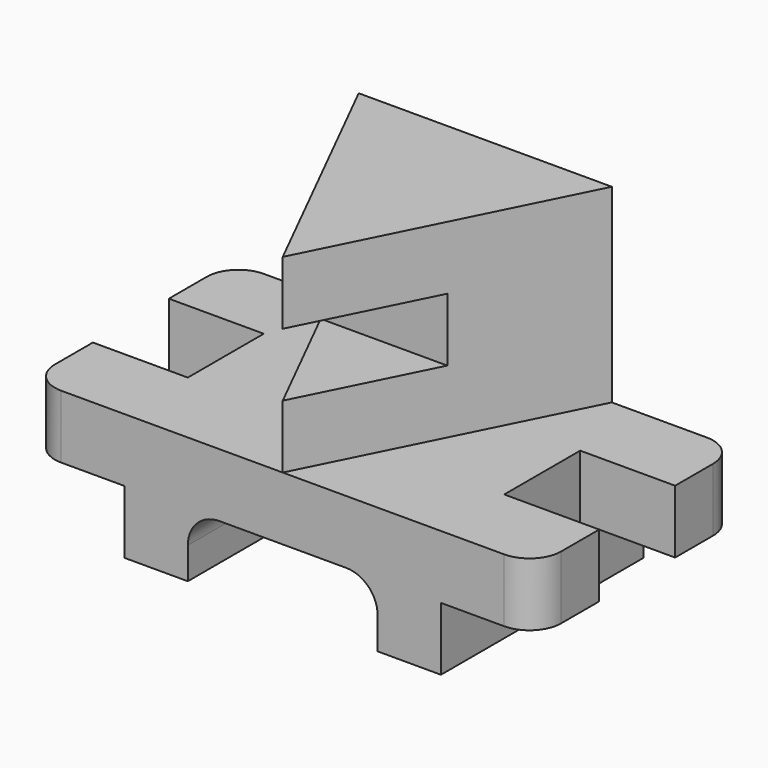
from build123d import *

# Parameters (mm, degrees)
F1_DEPTH       = 50.8
F2_W           = 76.2
F2_H           = 25.4
F3_DEPTH       = 101.601
F4_R           = 12.7
F5_R           = 12.7
F6_W           = 38.1
F6_H           = 25.4
F7_DEPTH       = 38.1
F8_W           = 38.1
F8_H           = 25.4
F9_DEPTH       = 38.1
F10_R          = 12.7
F11_W          = 101.6
F11_H          = 76.2
F12_DEPTH      = 50.8
F12_DEPTH_BACK = 50.8
F14_DEPTH      = 76.2
F15_W          = 50.8
F15_H          = 25.4
F16_DEPTH      = 101.601
F16_DEPTH_BACK = 356
F17_DEPTH      = 50.8


# Not quite as in the source:
# - an extrude ends at something that could not be found from the text; its depth is read off the source's solid


with BuildPart() as f1:
    # F0 (on Front) → F1 (new body, symmetric)
    with BuildSketch(Plane.XZ):
        Polygon((0, 25.4), (0, 0), (127, 0), (127, 25.4), (165.1, 25.4), (165.1, 50.8), (-38.1, 50.8), (-38.1, 25.4), align=None)
    extrude(amount=F1_DEPTH, both=True)

    # F2 (on face) → F3 (cut, through all)
    with BuildSketch(Plane.XZ.offset(50.8)):
        with Locations((63.5, 12.7)):
            Rectangle(F2_W, F2_H)
    extrude(amount=-F3_DEPTH, mode=Mode.SUBTRACT)

    # F4
    f4_edges = [f1.edges().sort_by_distance(p)[0] for p in [
        (25.4, 0, 25.4),
    ]]
    fillet(f4_edges, radius=F4_R)

    # F5
    f5_edges = [f1.edges().sort_by_distance(p)[0] for p in [
        (101.6, 0, 25.4),
    ]]
    fillet(f5_edges, radius=F5_R)

    # F6 (on face) → F7 (cut)
    with BuildSketch(Plane.YZ.offset(165.1)):
        with Locations((0, 38.1)):
            Rectangle(F6_W, F6_H)
    extrude(amount=-F7_DEPTH, mode=Mode.SUBTRACT)

    # F8 (on face) → F9 (cut)
    with BuildSketch(Plane(origin=(-38.1, 0, 0), x_dir=(0, -1, 0), z_dir=(-1, 0, 0))):
        with Locations((0, 38.1)):
            Rectangle(F8_W, F8_H)
    extrude(amount=-F9_DEPTH, mode=Mode.SUBTRACT)

    # F10
    f10_edges = [f1.edges().sort_by_distance(p)[0] for p in [
        (-38.1, -50.8, 38.1),
        (-38.1, 50.8, 38.1),
        (165.1, 50.8, 38.1),
        (165.1, -50.8, 38.1),
    ]]
    fillet(f10_edges, radius=F10_R)

    # F11 (on Front) → F12 (join, two sides)
    with BuildSketch(Plane.XZ) as f12_sk:
        with Locations((63.5, 88.9)):
            Rectangle(F11_W, F11_H)
    extrude(amount=-F12_DEPTH)
    extrude(f12_sk.sketch, amount=F12_DEPTH_BACK)

    # F13 (on face) → F14 (cut)
    with BuildSketch(Plane.XY.offset(127)):
        Polygon((63.5, -50.8), (12.7, 50.8), (12.7, -50.8), align=None)
        Polygon((114.3, 50.8), (63.5, -50.8), (114.3, -50.8), align=None)
    extrude(amount=-F14_DEPTH, mode=Mode.SUBTRACT)

    # F15 (on face) → F16 (cut, two sides)
    with BuildSketch(Plane(origin=(0, 50.8, 0), x_dir=(-1, 0, 0), z_dir=(0, 1, 0))) as f16_sk:
        with Locations((-63.5, 88.9)):
            Rectangle(F15_W, F15_H)
    extrude(amount=-F16_DEPTH, mode=Mode.SUBTRACT)
    extrude(f16_sk.sketch, amount=F16_DEPTH_BACK, mode=Mode.SUBTRACT)

    # F17 (add): a face of the model
    f17_faces = [f1.faces().sort_by_distance(p)[0] for p in [
        (38.1, 25.4, 88.9),
    ]]
    extrude(f17_faces, amount=F17_DEPTH)


solid = f1.part
